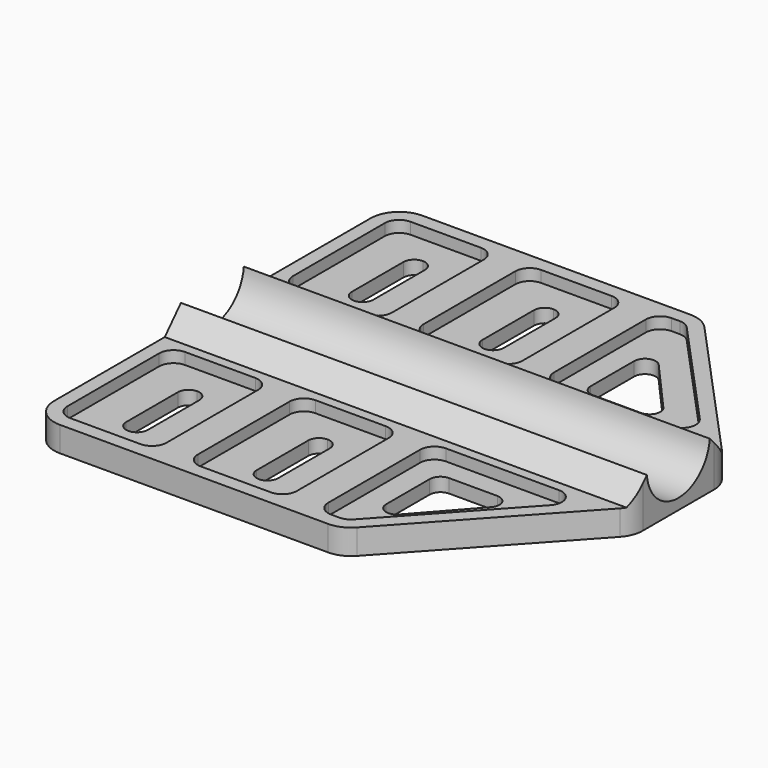
from build123d import *

# Parameters (mm, degrees)
F0_W         = 27.686
F0_H         = 19.685
F1_DEPTH     = 4.445
F4_DEPTH     = 82.55
F5_T4_DEPTH  = 82.55
F5_T9_DEPTH  = 82.55
F3_R         = 6.985
F6_DEPTH     = 101.6
F7_W         = 17.526
F7_H         = 25.4
F8_DEPTH     = 2.032
F9_R         = 2.54
F10_W        = 3.81
F10_H        = 15.24
F11_DEPTH    = 25.4
F12_R        = 1.90499
F13_T1_DEPTH = 29.845
F13_T3_DEPTH = 15.6401229428
F13_T5_DEPTH = 15.0634324568


# Not quite as in the source:
# - a fillet or chamfer that OpenCascade refuses, or shapes differently, is made with other operations: its cross-section is extruded or revolved along the edge and cut away or added
# - a fillet or chamfer is up to 0.001 mm smaller than in the source, because OpenCascade refuses the exact size


with BuildPart() as f1:
    # F0 (on Top) → F1 (new body)
    with BuildSketch(Plane.XY):
        Polygon((4.2753211141, 33.3069552488), (-50.5886788859, 33.3069552488), (-50.5886788859, -46.9570447512), (4.2753211141, -46.9570447512), (4.2753211141, -16.6675447512), (4.2753211141, 3.0174552488), align=None)
        Polygon((31.9613211141, 3.0174552488), (4.2753211141, 33.3069552488), (4.2753211141, 3.0174552488), align=None)
        with Locations((18.1183211141, -6.8250447512)):
            Rectangle(F0_W, F0_H)
        Polygon((4.2753211141, -16.6675447512), (4.2753211141, -46.9570447512), (31.9613211141, -16.6675447512), align=None)
    extrude(amount=F1_DEPTH)

    # F3 (on face) → F4 (join)
    with BuildSketch(Plane.YZ.offset(31.9613211141)):
        with BuildLine():
            Line((-1.4368910785, 4.445), (-12.2131984238, 4.445))
            ThreePointArc((-12.2131984238, 4.445), (-6.8250447512, 1.905), (-1.4368910785, 4.445))
        make_face()
        with BuildLine():
            ThreePointArc((-1.4368910785, 4.445), (-0.2513669981, 6.5284357306), (0.1599552488, 8.89))
            ThreePointArc((0.1599552488, 8.89), (-9.1866090205, 15.4636777531), (-12.2131984238, 4.445))
            Line((-12.2131984238, 4.445), (-1.4368910785, 4.445))
        make_face()
    extrude(amount=-F4_DEPTH)

    # F5: chamfer of 7.62 on 2 edges, made by hand


with BuildPart() as f5_tool2:
    # F5_s3 → F5_t4 (new body)
    with BuildSketch(Plane.YZ.offset(31.9613211141)):
        with BuildLine():
            Line((3.9242683255, 4.2209526948), (-0.0694446449, 8.550803314))
            Line((-0.0694446449, 8.550803314), (-0.2213483693, 8.5630922738))
            ThreePointArc((-0.2213483693, 8.5630922738), (-0.4679887951, 6.3855514916), (-1.554450795, 4.5419818182))
            Line((-1.554450795, 4.5419818182), (-1.4368910785, 4.2926))
            ThreePointArc((-1.4368910785, 4.2926), (1.2436886235, 4.2926), (3.9242683255, 4.0685526948))
            Line((3.9242683255, 4.0685526948), (3.9242683255, 4.2209526948))
        make_face()
    extrude(amount=-F5_T4_DEPTH)

    split(bisect_by=Plane(origin=(18.9157105891, 17.2898319012, 0), x_dir=(0, 0, 1), z_dir=(-0.7381168756, -0.6746728674, 0)), keep=Keep.TOP)


with BuildPart() as f1_1:
    add(f1.part)

    # F5_t1: union F5_tool2
    add(f5_tool2.part)


with BuildPart() as f5_tool7:
    # F5_s8 → F5_t9 (new body)
    with BuildSketch(Plane.YZ.offset(-50.5886788859)):
        with BuildLine():
            Line((-17.5743578278, 4.2209526948), (-13.5806448574, 8.550803314))
            Line((-13.5806448574, 8.550803314), (-13.4287411331, 8.5630922738))
            ThreePointArc((-13.4287411331, 8.5630922738), (-13.1821007073, 6.3855514916), (-12.0956387073, 4.5419818182))
            Line((-12.0956387073, 4.5419818182), (-12.2131984238, 4.2926))
            ThreePointArc((-12.2131984238, 4.2926), (-14.8937781258, 4.2926), (-17.5743578278, 4.0685526948))
            Line((-17.5743578278, 4.0685526948), (-17.5743578278, 4.2209526948))
        make_face()
    extrude(amount=F5_T9_DEPTH)

    split(bisect_by=Plane(origin=(25.7132835648, -23.5031271159, 0), x_dir=(0, 0, 1), z_dir=(-0.7381168756, 0.6746728674, 0)), keep=Keep.TOP)


with BuildPart() as f1_2:
    add(f1_1.part)

    # F5_t6: union F5_tool7
    add(f5_tool7.part)

    # F3 (on face) → F6 (cut)
    with BuildSketch(Plane.YZ.offset(31.9613211141)):
        with Locations((-6.8250447512, 8.89)):
            Circle(F3_R)
    extrude(amount=-F6_DEPTH, mode=Mode.SUBTRACT)

    # F7 (on face) → F8 (cut)
    with BuildSketch(Plane.XY.offset(4.445)):
        with Locations((-39.3872788859, -31.8059447512)):
            Rectangle(F7_W, F7_H)
        with Locations((-16.2732788859, -31.8186447512)):
            Rectangle(F7_W, F7_H)
        Polygon((26.4173608001, -19.1186447512), (-1.9222788859, -19.1186447512), (-1.9222788859, -44.5186447512), (3.2005893116, -44.5186447512), align=None)
        Polygon((3.2005893116, 30.8685552488), (-1.9222788859, 30.8685552488), (-1.9222788859, 5.4685552488), (26.4173608001, 5.4685552488), align=None)
        with Locations((-39.3872788859, 18.1558552488)):
            Rectangle(F7_W, F7_H)
        with Locations((-16.2732788859, 18.1685552488)):
            Rectangle(F7_W, F7_H)
    extrude(amount=-F8_DEPTH, mode=Mode.SUBTRACT)

    # F9
    f9_edges = [f1_2.edges().sort_by_distance(p)[0] for p in [
        (-48.150279, -19.105945, 3.429),
        (-48.150279, 30.855855, 3.429),
        (-25.036279, 30.868555, 3.429),
        (-1.922279, 30.868555, 3.429),
        (3.200589, 30.868555, 3.429),
        (-1.922279, -19.118645, 3.429),
        (-25.036279, -19.118645, 3.429),
        (-30.624279, 30.855855, 3.429),
        (-7.510279, 30.868555, 3.429),
        (26.417361, -19.118645, 3.429),
        (-7.510279, -19.118645, 3.429),
        (-30.624279, -19.105945, 3.429),
        (3.200589, -44.518645, 3.429),
        (-7.510279, -44.518645, 3.429),
        (-30.624279, -44.505945, 3.429),
        (-7.510279, 5.468555, 3.429),
        (-30.624279, 5.455855, 3.429),
        (-48.150279, 5.455855, 3.429),
        (-48.150279, -44.505945, 3.429),
        (-25.036279, -44.518645, 3.429),
        (-1.922279, -44.518645, 3.429),
        (-1.922279, 5.468555, 3.429),
        (-25.036279, 5.468555, 3.429),
        (26.417361, 5.468555, 3.429),
    ]]
    fillet(f9_edges, radius=F9_R)

    # F10 (on face) → F11 (cut)
    with BuildSketch(Plane.XY.offset(4.445)):
        with Locations((-39.3872788859, -31.8059447512)):
            Rectangle(F10_W, F10_H)
        with Locations((-16.2732788859, -31.8186447512)):
            Rectangle(F10_W, F10_H)
        Polygon((16.8492179688, -22.7416258461), (2.1748828364, -22.7416258461), (2.1748828364, -39.307281707), align=None)
        Polygon((16.8492179688, 9.0915363437), (2.1748828364, 25.6571922047), (2.1748828364, 9.0915363437), align=None)
        with Locations((-16.2732788859, 18.1685552488)):
            Rectangle(F10_W, F10_H)
        with Locations((-39.3872788859, 18.1558552488)):
            Rectangle(F10_W, F10_H)
    extrude(amount=-F11_DEPTH, mode=Mode.SUBTRACT)

    # F12 (radius 1.905 in the source; OpenCascade refuses exactly that, so slightly less here)
    f12_edges = [f1_2.edges().sort_by_distance(p)[0] for p in [
        (-41.292279, -24.185945, 1.2065),
        (-37.482279, -24.185945, 1.2065),
        (-14.368279, -24.198645, 1.2065),
        (16.849218, -22.741626, 1.2065),
        (-14.368279, 25.788555, 1.2065),
        (-37.482279, 25.775855, 1.2065),
        (-18.178279, -24.198645, 1.2065),
        (2.174883, -22.741626, 1.2065),
        (-18.178279, 25.788555, 1.2065),
        (-41.292279, 25.775855, 1.2065),
        (2.174883, 25.657192, 1.2065),
        (-41.292279, -39.425945, 1.2065),
        (-18.178279, -39.438645, 1.2065),
        (-41.292279, 10.535855, 1.2065),
        (-18.178279, 10.548555, 1.2065),
        (2.174883, 9.091536, 1.2065),
        (-14.368279, -39.438645, 1.2065),
        (-37.482279, -39.425945, 1.2065),
        (-14.368279, 10.548555, 1.2065),
        (-37.482279, 10.535855, 1.2065),
        (16.849218, 9.091536, 1.2065),
        (2.174883, -39.307282, 1.2065),
    ]]
    fillet(f12_edges, radius=F12_R)

    # F13: fillet of radius 5.08 on 6 edges, made by hand

    # F13_s2 → F13_t1 (cut)
    with BuildSketch(Plane.XY.offset(-12.7)):
        with BuildLine():
            ThreePointArc((-50.5886788859, -41.8770447512), (-49.1007813343, -45.4691471996), (-45.5086788859, -46.9570447512))
            Line((-45.5086788859, -46.9570447512), (-50.5886788859, -46.9570447512))
            Line((-50.5886788859, -46.9570447512), (-50.5886788859, -41.8770447512))
        make_face()
        with BuildLine():
            ThreePointArc((-45.5086788859, 33.3069552488), (-49.1007813343, 31.8190576973), (-50.5886788859, 28.2269552488))
            Line((-50.5886788859, 28.2269552488), (-50.5886788859, 33.3069552488))
            Line((-50.5886788859, 33.3069552488), (-45.5086788859, 33.3069552488))
        make_face()
    extrude(amount=F13_T1_DEPTH, mode=Mode.SUBTRACT)

    # F13_s4 → F13_t3 (cut)
    with BuildSketch(Plane.XY.offset(-5.5975614714)):
        with BuildLine():
            ThreePointArc((2.0362965256, -46.9570447512), (4.0851403599, -46.5255540759), (5.7859302534, -45.3043829175))
            Line((5.7859302534, -45.3043829175), (4.2753211141, -46.9570447512))
            Line((4.2753211141, -46.9570447512), (2.0362965256, -46.9570447512))
        make_face()
        with BuildLine():
            ThreePointArc((2.0362965256, 33.3069552488), (4.0851403599, 32.8754645736), (5.7859302534, 31.6542934152))
            Line((5.7859302534, 31.6542934152), (4.2753211141, 33.3069552488))
            Line((4.2753211141, 33.3069552488), (2.0362965256, 33.3069552488))
        make_face()
    extrude(amount=F13_T3_DEPTH, mode=Mode.SUBTRACT)

    # F13_s6 → F13_t5 (cut)
    with BuildSketch(Plane.XY.offset(-4.9296716098)):
        with BuildLine():
            ThreePointArc((31.9613211141, -14.6956761073), (31.6170649489, -16.5339172044), (30.630954842, -18.1230142736))
            Line((30.630954842, -18.1230142736), (31.9613211141, -16.6675447512))
            Line((31.9613211141, -16.6675447512), (31.9613211141, -14.6956761073))
        make_face()
        with BuildLine():
            ThreePointArc((30.630954842, 4.4729247713), (31.6170649489, 2.8838277021), (31.9613211141, 1.0455866049))
            Line((31.9613211141, 1.0455866049), (31.9613211141, 3.0174552488))
            Line((31.9613211141, 3.0174552488), (30.630954842, 4.4729247713))
        make_face()
    extrude(amount=F13_T5_DEPTH, mode=Mode.SUBTRACT)


solid = f1_2.part
